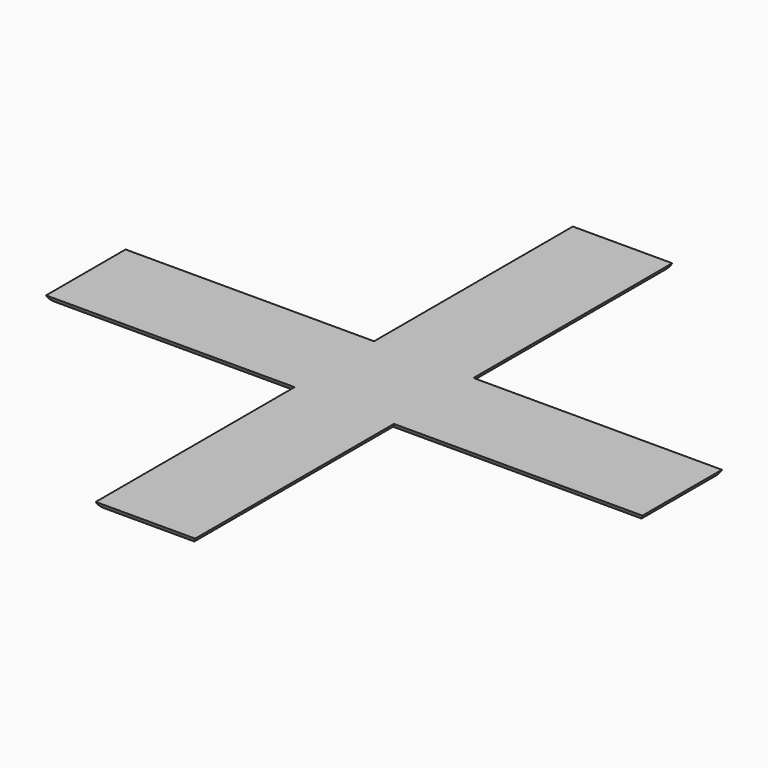
from build123d import *

# Parameters (mm, degrees)
F0_W         = 62.5
F0_H         = 25
F0_W_2       = 25
F0_H_2       = 62.5
F1_DEPTH     = 2
F2_T1_DEPTH  = 69.5710678119
F2_T3_DEPTH  = 69.5710678119
F2_T5_DEPTH  = 39.1421356237
F2_T7_DEPTH  = 69.5710678119
F2_T9_DEPTH  = 39.1421356237
F2_T11_DEPTH = 69.5710678119
F2_T17_DEPTH = 69.5710678119
F2_T21_DEPTH = 69.5710678119
F2_T28_DEPTH = 69.5710678119
F2_T32_DEPTH = 69.5710678119
F2_T39_DEPTH = 69.5710678119
F2_T43_DEPTH = 69.5710678119
F2_T50_DEPTH = 69.5710678119
F2_T54_DEPTH = 69.5710678119


# Not quite as in the source:
# - a fillet or chamfer that OpenCascade refuses, or shapes differently, is made with other operations: its cross-section is extruded or revolved along the edge and cut away or added
# - a feature names something its author has since deleted; it is built from what else it names


with BuildPart() as f1:
    # F0 (on Top) → F1 (new body)
    with BuildSketch(Plane.XY):
        with Locations((-43.75, 0)):
            Rectangle(F0_W, F0_H)
        Rectangle(F0_W_2, F0_H)
        with Locations((0, -43.75)):
            Rectangle(F0_W_2, F0_H_2)
        with Locations((0, 43.75)):
            Rectangle(F0_W_2, F0_H_2)
        with Locations((43.75, 0)):
            Rectangle(F0_W, F0_H)
    extrude(amount=F1_DEPTH)

    # F2: fillet of radius 3 on 12 edges, made by hand

    # F2_s2 → F2_t1 (cut)
    with BuildSketch(Plane.YZ.offset(-82.0710678119)):
        with BuildLine():
            ThreePointArc((-12.5, 2), (-11.4036236828, 0.5505102572), (-9.6715728753, 0))
            Line((-9.6715728753, 0), (-12.5, 0))
            Line((-12.5, 0), (-12.5, 2))
        make_face()
        with BuildLine():
            ThreePointArc((12.5, 2), (11.4036236828, 0.5505102572), (9.6715728753, 0))
            Line((9.6715728753, 0), (12.5, 0))
            Line((12.5, 0), (12.5, 2))
        make_face()
    extrude(amount=F2_T1_DEPTH, mode=Mode.SUBTRACT)

    # F2_s4 → F2_t3 (cut)
    with BuildSketch(Plane.XZ.offset(12.5)):
        with BuildLine():
            ThreePointArc((-12.5, 2), (-11.4036236828, 0.5505102572), (-9.6715728753, 0))
            Line((-9.6715728753, 0), (-12.5, 0))
            Line((-12.5, 0), (-12.5, 2))
        make_face()
        with BuildLine():
            ThreePointArc((12.5, 2), (11.4036236828, 0.5505102572), (9.6715728753, 0))
            Line((9.6715728753, 0), (12.5, 0))
            Line((12.5, 0), (12.5, 2))
        make_face()
    extrude(amount=F2_T3_DEPTH, mode=Mode.SUBTRACT)

    # F2_s6 → F2_t5 (cut)
    with BuildSketch(Plane.YZ.offset(-19.5710678119)):
        with BuildLine():
            ThreePointArc((-75, 2), (-73.9036236828, 0.5505102572), (-72.1715728753, 0))
            Line((-72.1715728753, 0), (-75, 0))
            Line((-75, 0), (-75, 2))
        make_face()
        with BuildLine():
            ThreePointArc((75, 2), (73.9036236828, 0.5505102572), (72.1715728753, 0))
            Line((72.1715728753, 0), (75, 0))
            Line((75, 0), (75, 2))
        make_face()
    extrude(amount=F2_T5_DEPTH, mode=Mode.SUBTRACT)

    # F2_s8 → F2_t7 (cut)
    with BuildSketch(Plane.YZ.offset(12.5)):
        with BuildLine():
            ThreePointArc((-12.5, 2), (-11.4036236828, 0.5505102572), (-9.6715728753, 0))
            Line((-9.6715728753, 0), (-12.5, 0))
            Line((-12.5, 0), (-12.5, 2))
        make_face()
        with BuildLine():
            ThreePointArc((12.5, 2), (11.4036236828, 0.5505102572), (9.6715728753, 0))
            Line((9.6715728753, 0), (12.5, 0))
            Line((12.5, 0), (12.5, 2))
        make_face()
    extrude(amount=F2_T7_DEPTH, mode=Mode.SUBTRACT)

    # F2_s10 → F2_t9 (cut)
    with BuildSketch(Plane.XZ.offset(-19.5710678119)):
        with BuildLine():
            ThreePointArc((75, 2), (73.9036236828, 0.5505102572), (72.1715728753, 0))
            Line((72.1715728753, 0), (75, 0))
            Line((75, 0), (75, 2))
        make_face()
        with BuildLine():
            ThreePointArc((-75, 2), (-73.9036236828, 0.5505102572), (-72.1715728753, 0))
            Line((-72.1715728753, 0), (-75, 0))
            Line((-75, 0), (-75, 2))
        make_face()
    extrude(amount=F2_T9_DEPTH, mode=Mode.SUBTRACT)

    # F2_s12 → F2_t11 (cut)
    with BuildSketch(Plane.XZ.offset(-82.0710678119)):
        with BuildLine():
            ThreePointArc((12.5, 2), (11.4036236828, 0.5505102572), (9.6715728753, 0))
            Line((9.6715728753, 0), (12.5, 0))
            Line((12.5, 0), (12.5, 2))
        make_face()
        with BuildLine():
            ThreePointArc((-12.5, 2), (-11.4036236828, 0.5505102572), (-9.6715728753, 0))
            Line((-9.6715728753, 0), (-12.5, 0))
            Line((-12.5, 0), (-12.5, 2))
        make_face()
    extrude(amount=F2_T11_DEPTH, mode=Mode.SUBTRACT)


with BuildPart() as f2_tool15:
    # F2_s16 → F2_t17 (new body)
    with BuildSketch(Plane.YZ.offset(-75)):
        with BuildLine():
            ThreePointArc((-12.5, 2), (-11.4036236828, 0.5505102572), (-9.6715728753, 0))
            Line((-9.6715728753, 0), (-12.5, 0))
            Line((-12.5, 0), (-12.5, 2))
        make_face()
    extrude(amount=F2_T17_DEPTH)

    split(bisect_by=Plane.YZ.offset(-12.5), keep=Keep.TOP)


with BuildPart() as f2_tool19:
    # F2_s20 → F2_t21 (new body)
    with BuildSketch(Plane.XZ.offset(5.4289321881)):
        with BuildLine():
            ThreePointArc((-12.5, 2), (-11.4036236828, 0.5505102572), (-9.6715728753, 0))
            Line((-9.6715728753, 0), (-12.5, 0))
            Line((-12.5, 0), (-12.5, 2))
        make_face()
    extrude(amount=F2_T21_DEPTH)

    split(bisect_by=Plane.XZ.offset(12.5), keep=Keep.BOTTOM)


with BuildPart() as f2_tool15_1:
    add(f2_tool15.part)

    # F2_t23: intersect F2_tool19
    add(f2_tool19.part, mode=Mode.INTERSECT)


with BuildPart() as f1_1:
    add(f1.part)

    # F2_t13: cut F2_tool15
    add(f2_tool15_1.part, mode=Mode.SUBTRACT)


with BuildPart() as f2_tool26:
    # F2_s27 → F2_t28 (new body)
    with BuildSketch(Plane.XZ.offset(75)):
        with BuildLine():
            ThreePointArc((12.5, 2), (11.4036236828, 0.5505102572), (9.6715728753, 0))
            Line((9.6715728753, 0), (12.5, 0))
            Line((12.5, 0), (12.5, 2))
        make_face()
    extrude(amount=-F2_T28_DEPTH)

    split(bisect_by=Plane.XZ.offset(12.5), keep=Keep.BOTTOM)


with BuildPart() as f2_tool30:
    # F2_s31 → F2_t32 (new body)
    with BuildSketch(Plane.YZ.offset(5.4289321881)):
        with BuildLine():
            ThreePointArc((-12.5, 2), (-11.4036236828, 0.5505102572), (-9.6715728753, 0))
            Line((-9.6715728753, 0), (-12.5, 0))
            Line((-12.5, 0), (-12.5, 2))
        make_face()
    extrude(amount=F2_T32_DEPTH)

    split(bisect_by=Plane.YZ.offset(12.5), keep=Keep.BOTTOM)


with BuildPart() as f2_tool26_1:
    add(f2_tool26.part)

    # F2_t34: intersect F2_tool30
    add(f2_tool30.part, mode=Mode.INTERSECT)


with BuildPart() as f1_2:
    add(f1_1.part)

    # F2_t24: cut F2_tool26
    add(f2_tool26_1.part, mode=Mode.SUBTRACT)


with BuildPart() as f2_tool37:
    # F2_s38 → F2_t39 (new body)
    with BuildSketch(Plane.YZ.offset(75)):
        with BuildLine():
            ThreePointArc((12.5, 2), (11.4036236828, 0.5505102572), (9.6715728753, 0))
            Line((9.6715728753, 0), (12.5, 0))
            Line((12.5, 0), (12.5, 2))
        make_face()
    extrude(amount=-F2_T39_DEPTH)

    split(bisect_by=Plane.YZ.offset(12.5), keep=Keep.BOTTOM)


with BuildPart() as f2_tool41:
    # F2_s42 → F2_t43 (new body)
    with BuildSketch(Plane.XZ.offset(-5.4289321881)):
        with BuildLine():
            ThreePointArc((12.5, 2), (11.4036236828, 0.5505102572), (9.6715728753, 0))
            Line((9.6715728753, 0), (12.5, 0))
            Line((12.5, 0), (12.5, 2))
        make_face()
    extrude(amount=-F2_T43_DEPTH)

    split(bisect_by=Plane.XZ.offset(-12.5), keep=Keep.TOP)


with BuildPart() as f2_tool37_1:
    add(f2_tool37.part)

    # F2_t45: intersect F2_tool41
    add(f2_tool41.part, mode=Mode.INTERSECT)


with BuildPart() as f1_3:
    add(f1_2.part)

    # F2_t35: cut F2_tool37
    add(f2_tool37_1.part, mode=Mode.SUBTRACT)


with BuildPart() as f2_tool48:
    # F2_s49 → F2_t50 (new body)
    with BuildSketch(Plane.XZ.offset(-75)):
        with BuildLine():
            ThreePointArc((-12.5, 2), (-11.4036236828, 0.5505102572), (-9.6715728753, 0))
            Line((-9.6715728753, 0), (-12.5, 0))
            Line((-12.5, 0), (-12.5, 2))
        make_face()
    extrude(amount=F2_T50_DEPTH)

    split(bisect_by=Plane.XZ.offset(-12.5), keep=Keep.TOP)


with BuildPart() as f2_tool52:
    # F2_s53 → F2_t54 (new body)
    with BuildSketch(Plane.YZ.offset(-5.4289321881)):
        with BuildLine():
            ThreePointArc((12.5, 2), (11.4036236828, 0.5505102572), (9.6715728753, 0))
            Line((9.6715728753, 0), (12.5, 0))
            Line((12.5, 0), (12.5, 2))
        make_face()
    extrude(amount=-F2_T54_DEPTH)

    split(bisect_by=Plane.YZ.offset(-12.5), keep=Keep.TOP)


with BuildPart() as f2_tool48_1:
    add(f2_tool48.part)

    # F2_t56: intersect F2_tool52
    add(f2_tool52.part, mode=Mode.INTERSECT)


with BuildPart() as f1_4:
    add(f1_3.part)

    # F2_t46: cut F2_tool48
    add(f2_tool48_1.part, mode=Mode.SUBTRACT)


solid = f1_4.part
